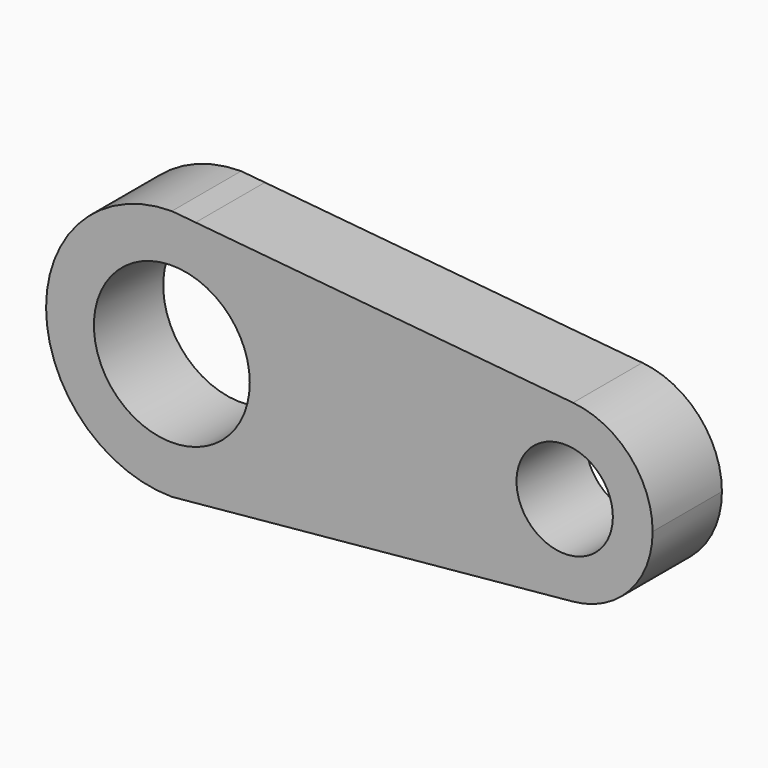
from build123d import *

# Parameters (mm, degrees)
F0_R     = 22.8532905428
F0_R_2   = 14.1278184646
F1_DEPTH = 25.4


with BuildPart() as f1:
    # F0 (on Front) → F1 (new body)
    with BuildSketch(Plane.XZ):
        with BuildLine():
            Line((6.9627707482, 36.2147105875), (0, 36.8779804142))
            ThreePointArc((0, 36.8779804142), (-36.8779804142, 0), (0, -36.8779804142))
            Line((0, -36.8779804142), (6.9627707482, -36.2147105875))
            ThreePointArc((6.9627707482, -36.2147105875), (28.4320098015, -23.4862993695), (36.8779804142, 0))
            ThreePointArc((36.8779804142, 0), (28.4320098015, 23.4862993695), (6.9627707482, 36.2147105875))
        make_face()
        Circle(F0_R, mode=Mode.SUBTRACT)
        with BuildLine():
            Line((117.6412233187, 25.6715402452), (6.9627707482, 36.2147105875))
            ThreePointArc((6.9627707482, 36.2147105875), (28.4320098015, 23.4862993695), (36.8779804142, 0))
            ThreePointArc((36.8779804142, 0), (28.4320098015, -23.4862993695), (6.9627707482, -36.2147105875))
            Line((6.9627707482, -36.2147105875), (117.6412233187, -25.6715402452))
            ThreePointArc((117.6412233187, -25.6715402452), (89.4080124161, 0), (117.6412233187, 25.6715402452))
        make_face()
        with BuildLine():
            ThreePointArc((140.9835197666, 0), (134.2754816057, 17.3485646526), (117.6412233187, 25.6715402452))
            ThreePointArc((117.6412233187, 25.6715402452), (89.4080124161, 0), (117.6412233187, -25.6715402452))
            ThreePointArc((117.6412233187, -25.6715402452), (134.2754816057, -17.3485646526), (140.9835197666, 0))
        make_face()
        with Locations((115.1957660913, 0)):
            Circle(F0_R_2, mode=Mode.SUBTRACT)
    extrude(amount=F1_DEPTH)


solid = f1.part
